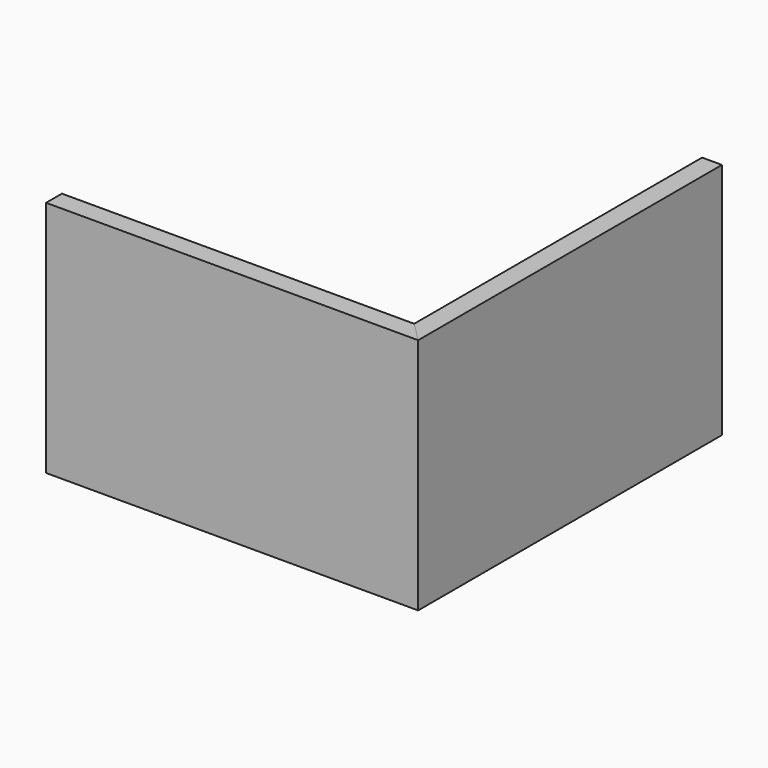
from build123d import *

# Parameters (mm, degrees)
F1_DEPTH   = 755
F3_W       = 1220
F3_H       = 780
F4_DEPTH   = 18
F5_SIZE    = 17.99999
F7_W       = 1245
F7_H       = 780
F8_DEPTH   = 18
F9_SIZE    = 17.99999
F11_W      = 65
F11_H      = 780
F12_DEPTH  = 18
F13_SIZE   = 17.99999
F15_W      = 65
F15_H      = 780
F16_DEPTH  = 18
F17_SIZE   = 17.99999
F22_DEPTH  = 18
F23_DEPTH  = 18
F24_SIZE   = 17.99999
F24_2_SIZE = 17.99999


# Not quite as in the source:
# - a fillet or chamfer is up to 0.001 mm smaller than in the source, because OpenCascade refuses the exact size


with BuildPart() as f1:
    # F0 (on Top) → F1 (new body)
    with BuildSketch(Plane.XY):
        Polygon((-1175, 45), (-1175, 0), (0, 0), (0, 1200), (-45, 1200), (-45, 45), align=None)
    extrude(amount=F1_DEPTH)


with BuildPart() as f4:
    # F3 (on offset) → F4 (new body)
    with BuildSketch(Plane.XZ.offset(20)):
        with Locations((-590, 390)):
            Rectangle(F3_W, F3_H)
    extrude(amount=-F4_DEPTH)

    # F5 (size 18 in the source; OpenCascade refuses exactly that, so slightly less here)
    f5_edges = [f4.edges().sort_by_distance(p)[0] for p in [
        (20, -2, 390),
        (-590, -2, 780),
        (-1200, -2, 390),
    ]]
    chamfer(f5_edges, length=F5_SIZE)


with BuildPart() as f8:
    # F7 (on offset) → F8 (new body)
    with BuildSketch(Plane.YZ.offset(20)):
        with Locations((602.5, 390)):
            Rectangle(F7_W, F7_H)
    extrude(amount=-F8_DEPTH)

    # F9 (size 18 in the source; OpenCascade refuses exactly that, so slightly less here)
    f9_edges = [f8.edges().sort_by_distance(p)[0] for p in [
        (2, -20, 390),
        (2, 602.5, 780),
        (2, 1225, 390),
    ]]
    chamfer(f9_edges, length=F9_SIZE)


with BuildPart() as f12:
    # F11 (on face) → F12 (new body)
    with BuildSketch(Plane.YZ.offset(-1200)):
        with Locations((12.5, 390)):
            Rectangle(F11_W, F11_H)
    extrude(amount=F12_DEPTH)

    # F13 (size 18 in the source; OpenCascade refuses exactly that, so slightly less here)
    f13_edges = [f12.edges().sort_by_distance(p)[0] for p in [
        (-1182, 12.5, 780),
        (-1182, -20, 390),
    ]]
    chamfer(f13_edges, length=F13_SIZE)


with BuildPart() as f16:
    # F15 (on face) → F16 (new body)
    with BuildSketch(Plane.XZ.offset(-1225)):
        with Locations((-12.5, 390)):
            Rectangle(F15_W, F15_H)
    extrude(amount=F16_DEPTH)

    # F17 (size 18 in the source; OpenCascade refuses exactly that, so slightly less here)
    f17_edges = [f16.edges().sort_by_distance(p)[0] for p in [
        (20, 1207, 390),
        (-12.5, 1207, 780),
    ]]
    chamfer(f17_edges, length=F17_SIZE)


with BuildPart() as f22:
    # F21 (on face) → F22 (new body)
    with BuildSketch(Plane(origin=(0, 0, 780), x_dir=(1, 0, 0), z_dir=(0, 0, -1))):
        Polygon((-1200, 20), (-1200, -45), (-45, -45), (20, 20), align=None)
    extrude(amount=F22_DEPTH)

    # F24 (size 18 in the source; OpenCascade refuses exactly that, so slightly less here)
    f24_edges = [f22.edges().sort_by_distance(p)[0] for p in [
        (-1200, 12.5, 762),
        (-590, -20, 762),
    ]]
    chamfer(f24_edges, length=F24_SIZE)


with BuildPart() as f23:
    # F19 (on face) → F23 (new body)
    with BuildSketch(Plane.XY.offset(780)):
        Polygon((-45, 45), (20, -20), (20, 1225), (-45, 1225), align=None)
    extrude(amount=-F23_DEPTH)

    # F24#2 (size 18 in the source; OpenCascade refuses exactly that, so slightly less here)
    f24_2_edges = [f23.edges().sort_by_distance(p)[0] for p in [
        (20, 602.5, 762),
        (-12.5, 1225, 762),
    ]]
    chamfer(f24_2_edges, length=F24_2_SIZE)


solid = Compound([f1.part, f4.part, f8.part, f12.part, f16.part, f22.part, f23.part])
